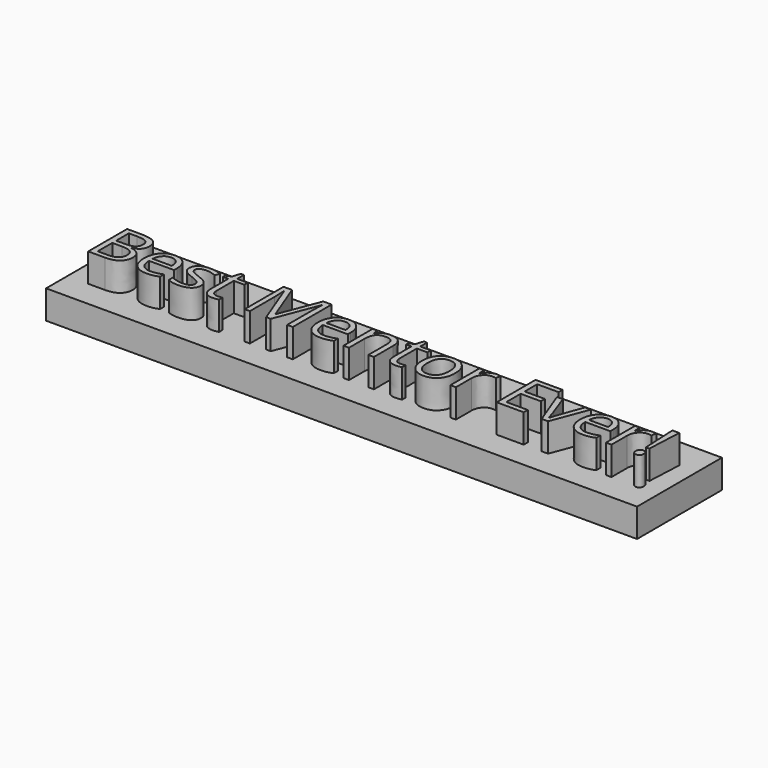
from build123d import *

# Parameters (mm, degrees)
F0_W         = 103.5954877734
F0_H         = 18.5977863148
F1_DEPTH     = 5
F2_TEXT_SIZE = 11.9292309844
F3_DEPTH     = 5


# Not quite as in the source:
# - Text() gives the source's letters only with a copy of the font that has no kerning and outlines rounded to 1/6400 em; it was checked with that copy


with BuildPart() as f1:
    # F0 (on Top) → F1 (new body)
    with BuildSketch(Plane.XY):
        with Locations((12.568037957, 4.648538772)):
            Rectangle(F0_W, F0_H)
    extrude(amount=F1_DEPTH)

    # F2 (on face) → F3 (join)
    with BuildSketch(Plane.XY.offset(5)):
        with Locations((-36.730810461, 0)):
            Text('Best Mentor Ever!', F2_TEXT_SIZE, font='Open Sans', text_align=(TextAlign.LEFT, TextAlign.BOTTOM))
    extrude(amount=F3_DEPTH)


solid = f1.part
